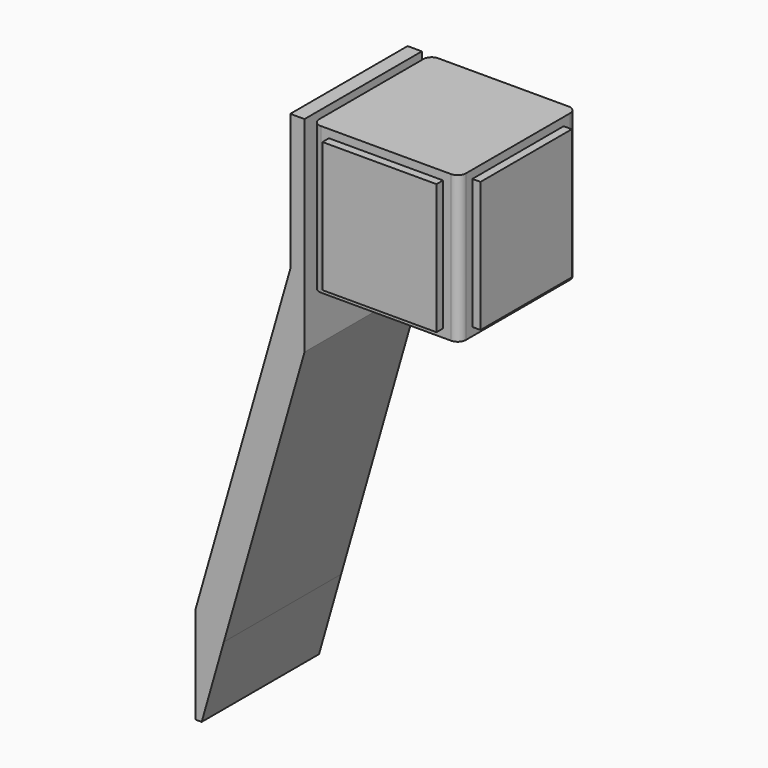
from build123d import *

# Parameters (mm, degrees)
F1_DEPTH  = 457.2
F2_W      = 355.6
F2_H      = 406.4
F3_DEPTH  = 25.4
F4_W      = 355.6
F4_H      = 406.4
F5_DEPTH  = 25.4
F6_W      = 355.6
F6_H      = 406.4
F7_DEPTH  = 25.4
F8_W      = 355.6
F8_H      = 406.4
F9_DEPTH  = 25.4
F11_DEPTH = 228.6


# Not quite as in the source:
# - a feature of the source that left no trace in its solid (it failed there, or was rolled back) is left out


with BuildPart() as f1:
    # F0 (on Top) → F1 (new body)
    with BuildSketch(Plane.XY):
        with BuildLine():
            ThreePointArc((-228.6, -203.2), (-221.1605122421, -221.1605122421), (-203.2, -228.6))
            Line((-203.2, -228.6), (203.2, -228.6))
            ThreePointArc((203.2, -228.6), (221.1605122421, -221.1605122421), (228.6, -203.2))
            Line((228.6, -203.2), (228.6, 203.2))
            ThreePointArc((228.6, 203.2), (221.1605122421, 221.1605122421), (203.2, 228.6))
            Line((203.2, 228.6), (-203.2, 228.6))
            ThreePointArc((-203.2, 228.6), (-221.1605122421, 221.1605122421), (-228.6, 203.2))
            Line((-228.6, 203.2), (-228.6, -203.2))
        make_face()
    extrude(amount=F1_DEPTH)

    # F2 (on face) → F3 (join)
    with BuildSketch(Plane.YZ.offset(228.6)):
        with Locations((0, 228.6)):
            Rectangle(F2_W, F2_H)
    extrude(amount=F3_DEPTH)

    # F4 (on face) → F5 (join)
    with BuildSketch(Plane.XZ.offset(228.6)):
        with Locations((0, 228.6)):
            Rectangle(F4_W, F4_H)
    extrude(amount=F5_DEPTH)

    # F6 (on face) → F7 (join)
    with BuildSketch(Plane(origin=(-228.6, 0, 0), x_dir=(0, -1, 0), z_dir=(-1, 0, 0))):
        with Locations((0, 228.6)):
            Rectangle(F6_W, F6_H)
    extrude(amount=F7_DEPTH)

    # F8 (on face) → F9 (join)
    with BuildSketch(Plane(origin=(0, 228.6, 0), x_dir=(-1, 0, 0), z_dir=(0, 1, 0))):
        with Locations((0, 228.6)):
            Rectangle(F8_W, F8_H)
    extrude(amount=F9_DEPTH)


with BuildPart() as f11:
    # F10 (on Front) → F11 (new body, symmetric)
    with BuildSketch(Plane.XZ):
        Polygon((-254, -179.6818675809), (-254, 459.6689861676), (-298.45, 459.6689861676), (-298.45, 33.9028166904), (-593.6153675181, -995.4611493138), (-593.6153675181, -1298.9769535385), (-574.5653675181, -1298.9769535385), (-505.5949514657, -1057.0977353197), align=None)
    extrude(amount=F11_DEPTH, both=True)


solid = Compound([f1.part, f11.part])
